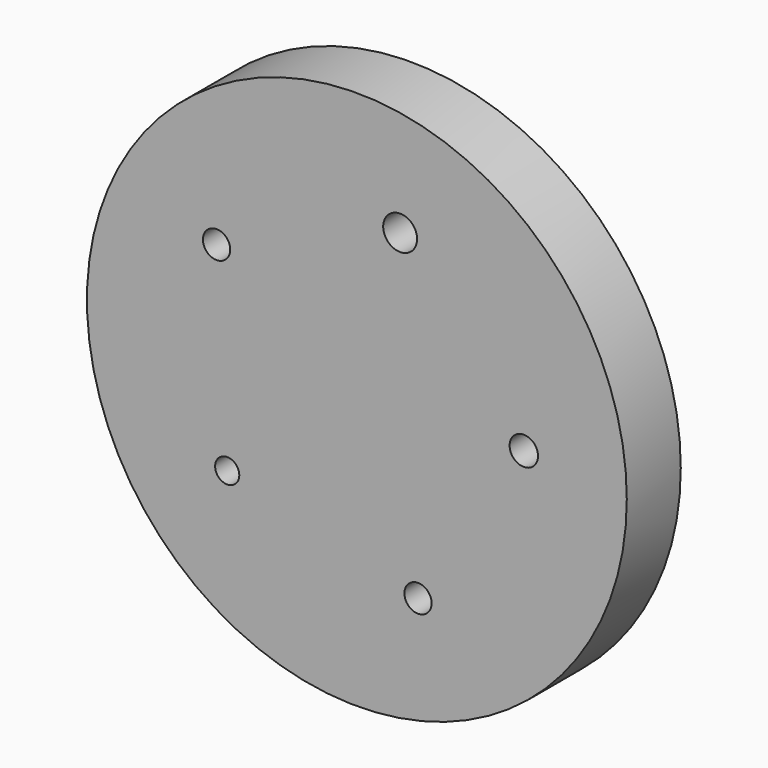
from build123d import *

# Parameters (mm, degrees)
F1_R     = 101.6
F1_R_2   = 4.5494653294
F1_R_3   = 5.1204654318
F1_R_4   = 5.1430144974
F1_R_5   = 5.3478696025
F1_R_6   = 6.3874946109
F3_DEPTH = 25.4


# Not quite as in the source:
# - the program builds the solid bodies; features that only make, move or delete a surface that nothing else refers to are left out


with BuildPart() as f3:
    # F1 (on face) → F3 (new body)
    with BuildSketch(Plane.XZ):
        with Locations((-34.2702679336, 12.4070197344)):
            Circle(F1_R)
        with Locations((-83.0803439021, -27.0566623658)):
            Circle(F1_R_2, mode=Mode.SUBTRACT)
        with Locations((-11.2562878057, -45.9673032165)):
            Circle(F1_R_3, mode=Mode.SUBTRACT)
        with Locations((-87.0806723833, 46.585727483)):
            Circle(F1_R_4, mode=Mode.SUBTRACT)
        with Locations((28.565146029, 15.8559419215)):
            Circle(F1_R_5, mode=Mode.SUBTRACT)
        with Locations((-17.984110862, 72.9515254498)):
            Circle(F1_R_6, mode=Mode.SUBTRACT)
    extrude(amount=F3_DEPTH)


solid = f3.part
